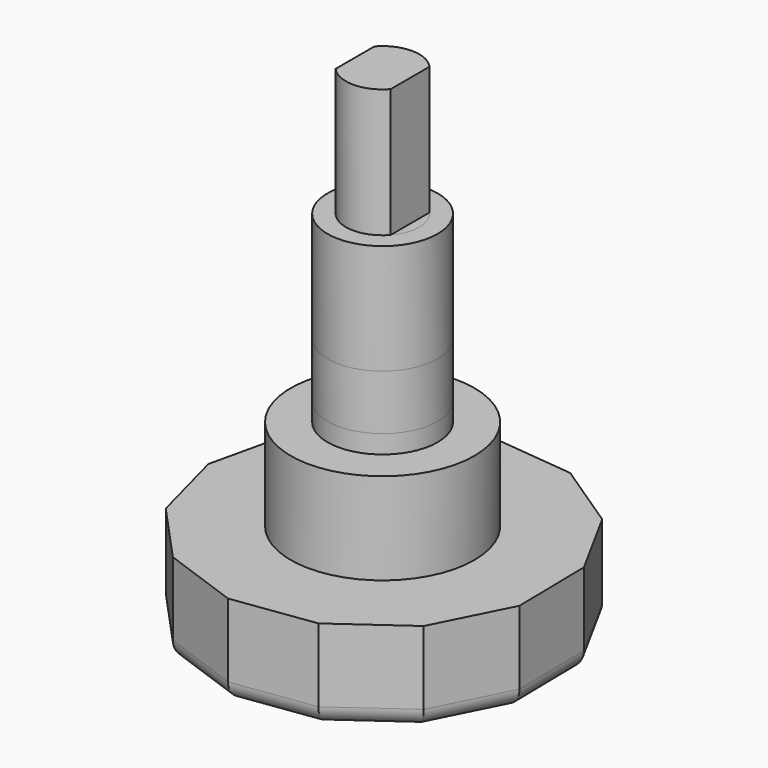
from build123d import *

# Parameters (mm, degrees)
F0_R           = 3
F1_DEPTH       = 9
F1_FACE_R      = 3
F2_DEPTH       = 6
F3_R           = 2
F4_DEPTH       = 7
F3_R_2         = 3
F5_DEPTH       = 7
F7_DEPTH       = 7
F8_R           = 5.0059936483
F9_DEPTH       = 5
F10_R          = 1
F8_R_2         = 3
F12_DEPTH      = 5
F12_DEPTH_BACK = 5
F13_DEPTH      = 1


with BuildPart() as f1:
    # F0 (on Top) → F1 (new body)
    with BuildSketch(Plane.XY):
        Circle(F0_R)
    extrude(amount=F1_DEPTH)

    # F0 (on Top) + F1_face (on face) → F2 (join)
    with BuildSketch(Plane.XY):
        Circle(F0_R)
    with BuildSketch(Plane.XY.offset(9)):
        Circle(F1_FACE_R)
    extrude(amount=-F2_DEPTH)

    # F3 (on face) → F4 (join)
    with BuildSketch(Plane.XY.offset(9)):
        Circle(F3_R)
    extrude(amount=F4_DEPTH)

    # F3 (on face) → F5 (cut)
    with BuildSketch(Plane.XY.offset(9)):
        Circle(F3_R_2)
        Circle(F3_R, mode=Mode.SUBTRACT)
    extrude(amount=F5_DEPTH, mode=Mode.SUBTRACT)

    # F6 (on face) → F7 (cut)
    with BuildSketch(Plane.XY.offset(16)):
        with BuildLine():
            Line((-1.5, -1.3228756555), (-1.5, 1.3228756555))
            ThreePointArc((-1.5, 1.3228756555), (-2, 0), (-1.5, -1.3228756555))
        make_face()
        with BuildLine():
            ThreePointArc((2, 0), (1.8708286934, 0.7071067812), (1.5, 1.3228756555))
            Line((1.5, 1.3228756555), (1.5, -1.3228756555))
            ThreePointArc((1.5, -1.3228756555), (1.8708286934, -0.7071067812), (2, 0))
        make_face()
    extrude(amount=-F7_DEPTH, mode=Mode.SUBTRACT)

    # F8 (on face) → F12 (join, two sides)
    with BuildSketch(Plane(origin=(0, 0, -6), x_dir=(1, 0, 0), z_dir=(0, 0, -1))) as f12_sk:
        Circle(F8_R)
        Circle(F8_R_2, mode=Mode.SUBTRACT)
    extrude(amount=-F12_DEPTH)
    extrude(f12_sk.sketch, amount=F12_DEPTH_BACK)


with BuildPart() as f9:
    # F8 (on face) → F9 (new body)
    with BuildSketch(Plane(origin=(0, 0, -6), x_dir=(1, 0, 0), z_dir=(0, 0, -1))):
        Polygon((-5.1929931591, 7.8022541948), (-8.2240554024, 4.4952487372), (-9.3710856636, 0.1584359675), (-8.3713131331, -4.214672573), (-5.4537736491, -7.6222504193), (-1.2868403472, -9.2836625527), (3.1748925702, -8.8182994754), (6.9092958614, -6.3327702604), (9.0608627367, -2.3964796969), (9.1366951543, 2.0888154845), (7.1194208212, 6.0955882113), (3.4711729762, 8.7059351387), (-0.9722787654, 9.3218572438), align=None)
        Circle(F8_R, mode=Mode.SUBTRACT)
    extrude(amount=F9_DEPTH)

    # F10
    f10_edges = [f9.edges().sort_by_distance(p)[0] for p in [
        (-6.708524, -6.148751, -11),
        (-3.082636, -8.562056, -11),
        (1.249447, -9.013896, -11),
        (5.295297, -7.400762, -11),
        (8.128058, -4.092202, -11),
        (9.098779, 0.153832, -11),
        (7.985079, 4.364625, -11),
        (5.042094, 7.575535, -11),
        (0.944026, 9.050981, -11),
        (-3.370307, 8.452956, -11),
        (-6.912543, 5.918461, -11),
        (-8.871199, 2.028118, -11),
        (-8.797571, -2.326842, -11),
    ]]
    fillet(f10_edges, radius=F10_R)

    # F11 (on face) → F13 (cut)
    with BuildSketch(Plane(origin=(0, 0, -11), x_dir=(1, 0, 0), z_dir=(0, 0, -1))):
        Polygon((7.7285151929, 0), (6.0742069036, 0.9805487934), (6.0742069036, -0.9805487934), align=None)
    extrude(amount=-F13_DEPTH, mode=Mode.SUBTRACT)


solid = Compound([f1.part, f9.part])
